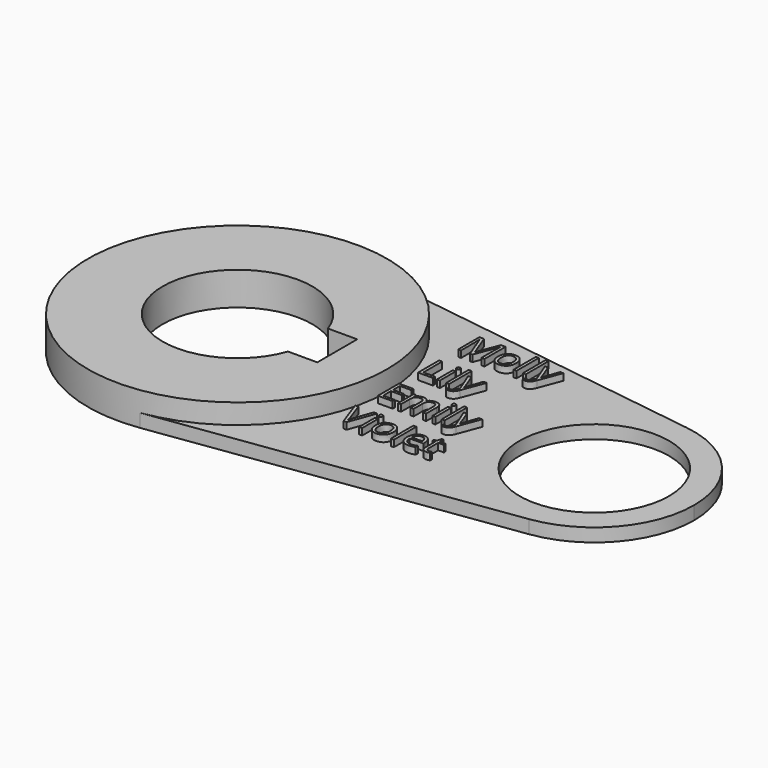
from build123d import *

# Parameters (mm, degrees)
F0_R         = 14.2875
F1_DEPTH     = 2.54
F2_DEPTH     = 6.35
F3_TEXT_SIZE = 7.0555555556
F4_DEPTH     = 1.27


# Not quite as in the source:
# - Text() gives the source's letters only with a copy of the font that has no kerning and outlines rounded to 1/6400 em; it was checked with that copy


with BuildPart() as f1:
    # F0 (on Top) → F1 (new body)
    with BuildSketch(Plane.XY):
        with BuildLine():
            ThreePointArc((3.9942349364, -28.2944643397), (21.5715772292, -18.7402689641), (28.575, 0))
            ThreePointArc((28.575, 0), (21.5715772292, 18.7402689641), (3.9942349364, 28.2944643397))
            ThreePointArc((3.9942349364, 28.2944643397), (-28.575, 0), (3.9942349364, -28.2944643397))
        make_face()
        with BuildLine():
            ThreePointArc((-13.4703841816, 4.7625), (0, 14.2875), (13.4703841816, 4.7625))
            Line((13.4703841816, 4.7625), (19.05, 4.7625))
            Line((19.05, 4.7625), (19.05, -4.7625))
            Line((19.05, -4.7625), (13.4703841816, -4.7625))
            ThreePointArc((13.4703841816, -4.7625), (0, -14.2875), (-13.4703841816, -4.7625))
            Line((-13.4703841816, -4.7625), (-19.05, -4.7625))
            Line((-19.05, -4.7625), (-19.05, 4.7625))
            Line((-19.05, 4.7625), (-13.4703841816, 4.7625))
        make_face(mode=Mode.SUBTRACT)
        with BuildLine():
            ThreePointArc((-13.4703841816, -4.7625), (-14.2875, 0), (-13.4703841816, 4.7625))
            Line((-13.4703841816, 4.7625), (-19.05, 4.7625))
            Line((-19.05, 4.7625), (-19.05, -4.7625))
            Line((-19.05, -4.7625), (-13.4703841816, -4.7625))
        make_face()
        with BuildLine():
            ThreePointArc((3.9942349364, 28.2944643397), (21.5715772292, 18.7402689641), (28.575, 0))
            ThreePointArc((28.575, 0), (21.5715772292, -18.7402689641), (3.9942349364, -28.2944643397))
            Line((3.9942349364, -28.2944643397), (70.8052534017, -18.8629762265))
            ThreePointArc((70.8052534017, -18.8629762265), (49.0924301108, 0), (70.8052534017, 18.8629762265))
            Line((70.8052534017, 18.8629762265), (3.9942349364, 28.2944643397))
        make_face()
        with BuildLine():
            ThreePointArc((87.1924301108, 0), (82.5234815969, 12.4935126427), (70.8052534017, 18.8629762265))
            ThreePointArc((70.8052534017, 18.8629762265), (49.0924301108, 0), (70.8052534017, -18.8629762265))
            ThreePointArc((70.8052534017, -18.8629762265), (82.5234815969, -12.4935126427), (87.1924301108, 0))
        make_face()
        with Locations((68.1424301108, 0)):
            Circle(F0_R, mode=Mode.SUBTRACT)
    extrude(amount=F1_DEPTH)

    # F0 (on Top) → F2 (join)
    with BuildSketch(Plane.XY):
        with BuildLine():
            ThreePointArc((3.9942349364, -28.2944643397), (21.5715772292, -18.7402689641), (28.575, 0))
            ThreePointArc((28.575, 0), (21.5715772292, 18.7402689641), (3.9942349364, 28.2944643397))
            ThreePointArc((3.9942349364, 28.2944643397), (-28.575, 0), (3.9942349364, -28.2944643397))
        make_face()
        with BuildLine():
            ThreePointArc((-13.4703841816, 4.7625), (0, 14.2875), (13.4703841816, 4.7625))
            Line((13.4703841816, 4.7625), (19.05, 4.7625))
            Line((19.05, 4.7625), (19.05, -4.7625))
            Line((19.05, -4.7625), (13.4703841816, -4.7625))
            ThreePointArc((13.4703841816, -4.7625), (0, -14.2875), (-13.4703841816, -4.7625))
            Line((-13.4703841816, -4.7625), (-19.05, -4.7625))
            Line((-19.05, -4.7625), (-19.05, 4.7625))
            Line((-19.05, 4.7625), (-13.4703841816, 4.7625))
        make_face(mode=Mode.SUBTRACT)
        with BuildLine():
            ThreePointArc((-13.4703841816, -4.7625), (-14.2875, 0), (-13.4703841816, 4.7625))
            Line((-13.4703841816, 4.7625), (-19.05, 4.7625))
            Line((-19.05, 4.7625), (-19.05, -4.7625))
            Line((-19.05, -4.7625), (-13.4703841816, -4.7625))
        make_face()
    extrude(amount=F2_DEPTH)

    # F3 (on face) → F4 (join)
    with BuildSketch(Plane.XY.offset(2.54)):
        with Locations((29.1051763208, 15.4590316363)):
            Text('Molly', F3_TEXT_SIZE, font='Open Sans', text_align=(TextAlign.LEFT, TextAlign.BOTTOM))
        with Locations((29.1051763208, 5.8634760807)):
            Text('Lily', F3_TEXT_SIZE, font='Open Sans', text_align=(TextAlign.LEFT, TextAlign.BOTTOM))
        with Locations((29.1051763208, -3.7320794748)):
            Text('Emily', F3_TEXT_SIZE, font='Open Sans', text_align=(TextAlign.LEFT, TextAlign.BOTTOM))
        with Locations((29.1051763208, -13.3276350304)):
            Text('Violet', F3_TEXT_SIZE, font='Open Sans', text_align=(TextAlign.LEFT, TextAlign.BOTTOM))
    extrude(amount=F4_DEPTH)


solid = f1.part
